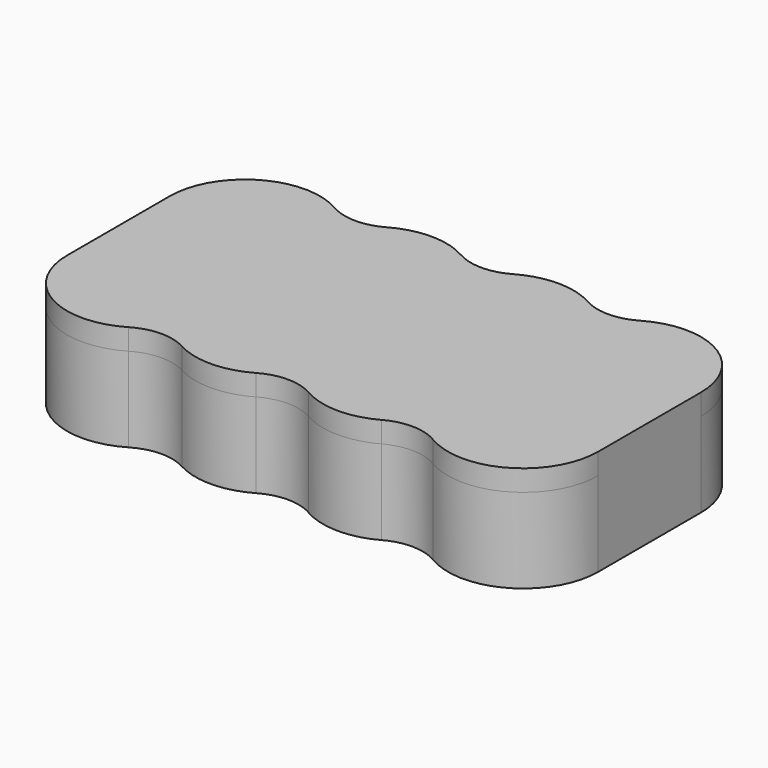
from build123d import *

# Parameters (mm, degrees)
F1_DEPTH  = 8
F2_R      = 5
F3_R      = 5.1
F5_DEPTH  = 2
F6_R      = 2
F7_DEPTH  = 1.5
F8_R      = 1.49999
F9_R      = 2
F10_DEPTH = 1.5
F11_R     = 1.49999


# Not quite as in the source:
# - a fillet or chamfer is up to 0.001 mm smaller than in the source, because OpenCascade refuses the exact size


with BuildPart() as f1:
    # F0 (on Top) → F1 (new body)
    with BuildSketch(Plane.XY):
        with BuildLine():
            ThreePointArc((0, 9.7960505792), (-5.9794748492, 13.0999703322), (-11.9779520569, 9.830677382))
            ThreePointArc((-11.9779520569, 9.830677382), (-19.9562029041, 12.8948954194), (-25.1, 6.0697016347))
            Line((-25.1, 6.0697016347), (-25.1, -6.0697016347))
            ThreePointArc((-25.1, -6.0697016347), (-19.9296547743, -12.9024486996), (-11.9488922671, -9.7837419151))
            ThreePointArc((-11.9488922671, -9.7837419151), (-5.9300692346, -12.9669396851), (0, -9.6213070677))
            ThreePointArc((0, -9.6213070677), (5.9300692346, -12.9669396851), (11.9488922671, -9.7837419151))
            ThreePointArc((11.9488922671, -9.7837419151), (19.9296547743, -12.9024486996), (25.1, -6.0697016347))
            Line((25.1, -6.0697016347), (25.1, 6.0697016347))
            ThreePointArc((25.1, 6.0697016347), (19.9562029041, 12.8948954194), (11.9779520569, 9.830677382))
            ThreePointArc((11.9779520569, 9.830677382), (5.9794748492, 13.0999703322), (0, 9.7960505792))
        make_face()
        with BuildLine():
            ThreePointArc((-24.1, 6.0697016347), (-18.5343432382, 12.1462530666), (-11.9936139988, 7.1342800509))
            ThreePointArc((-11.9936139988, 7.1342800509), (-5.9825651004, 12.0999750839), (0, 7.1))
            ThreePointArc((0, 7.1), (5.9825651004, 12.0999750839), (11.9936139988, 7.1342800509))
            ThreePointArc((11.9936139988, 7.1342800509), (18.5343432382, 12.1462530666), (24.1, 6.0697016347))
            Line((24.1, 6.0697016347), (24.1, -6.0697016347))
            ThreePointArc((24.1, -6.0697016347), (18.5343432382, -12.1462530666), (11.9936139988, -7.1342800509))
            ThreePointArc((11.9936139988, -7.1342800509), (5.8623077698, -11.9653833554), (0, -6.8111789722))
            ThreePointArc((0, -6.8111789722), (-5.8623077698, -11.9653833554), (-11.9936139988, -7.1342800509))
            ThreePointArc((-11.9936139988, -7.1342800509), (-18.5343432382, -12.1462530666), (-24.1, -6.0697016347))
            Line((-24.1, -6.0697016347), (-24.1, 6.0697016347))
        make_face(mode=Mode.SUBTRACT)
    extrude(amount=F1_DEPTH)

    # F2
    f2_edges = [f1.edges().sort_by_distance(p)[0] for p in [
        (-11.948892, -9.783742, 4),
        (0, -9.621307, 4),
        (11.948892, -9.783742, 4),
        (-11.977952, 9.830677, 4),
        (0, 9.796051, 4),
        (11.977952, 9.830677, 4),
    ]]
    fillet(f2_edges, radius=F2_R)

    # F3
    f3_edges = [f1.edges().sort_by_distance(p)[0] for p in [
        (-11.993614, -7.13428, 4),
        (0, -6.811179, 4),
        (11.993614, -7.13428, 4),
        (11.993614, 7.13428, 4),
        (0, 7.1, 4),
        (-11.993614, 7.13428, 4),
    ]]
    fillet(f3_edges, radius=F3_R)

    # F4 (on face) → F5 (join)
    with BuildSketch(Plane.XY.offset(8)):
        with BuildLine():
            ThreePointArc((-9.4848491067, 12.1859378193), (-11.9680100538, 11.5423164018), (-14.4435267926, 12.2147401477))
            ThreePointArc((-14.4435267926, 12.2147401477), (-21.5467619195, 12.2203503717), (-25.1, 6.0697016347))
            Line((-25.1, 6.0697016347), (-25.1, -6.0697016347))
            ThreePointArc((-25.1, -6.0697016347), (-21.5163446166, -12.2377905233), (-14.3830082993, -12.179314637))
            ThreePointArc((-14.3830082993, -12.179314637), (-11.9202167891, -11.4825711508), (-9.4353135356, -12.0957997614))
            ThreePointArc((-9.4353135356, -12.0957997614), (-5.9534768613, -12.9672192968), (-2.4903217652, -12.0242901298))
            ThreePointArc((-2.4903217652, -12.0242901298), (0, -11.3599904776), (2.4903217652, -12.0242901298))
            ThreePointArc((2.4903217652, -12.0242901298), (5.9534768613, -12.9672192968), (9.4353135356, -12.0957997614))
            ThreePointArc((9.4353135356, -12.0957997614), (11.9202167891, -11.4825711508), (14.3830082993, -12.179314637))
            ThreePointArc((14.3830082993, -12.179314637), (21.5163446166, -12.2377905233), (25.1, -6.0697016347))
            Line((25.1, -6.0697016347), (25.1, 6.0697016347))
            ThreePointArc((25.1, 6.0697016347), (21.5467619195, 12.2203503717), (14.4435267926, 12.2147401477))
            ThreePointArc((14.4435267926, 12.2147401477), (11.9680100538, 11.5423164018), (9.4848491067, 12.1859378193))
            ThreePointArc((9.4848491067, 12.1859378193), (5.9794143891, 13.0999701572), (2.479338843, 12.1656260848))
            ThreePointArc((2.479338843, 12.1656260848), (0, 11.5076162853), (-2.479338843, 12.1656260848))
            ThreePointArc((-2.479338843, 12.1656260848), (-5.9794143891, 13.0999701572), (-9.4848491067, 12.1859378193))
        make_face()
    extrude(amount=F5_DEPTH)

    # F6 (on face) → F7 (join)
    with BuildSketch(Plane.YZ.offset(-24.1)):
        with Locations((0, 4)):
            Circle(F6_R)
    extrude(amount=F7_DEPTH)

    # F8 (radius 1.5 in the source; OpenCascade refuses exactly that, so slightly less here)
    f8_edges = [f1.edges().sort_by_distance(p)[0] for p in [
        (-22.6, -2, 4),
    ]]
    fillet(f8_edges, radius=F8_R)

    # F9 (on face) → F10 (join)
    with BuildSketch(Plane(origin=(24.1, 0, 0), x_dir=(0, -1, 0), z_dir=(-1, 0, 0))):
        with Locations((0, 4)):
            Circle(F9_R)
    extrude(amount=F10_DEPTH)

    # F11 (radius 1.5 in the source; OpenCascade refuses exactly that, so slightly less here)
    f11_edges = [f1.edges().sort_by_distance(p)[0] for p in [
        (22.6, 2, 4),
    ]]
    fillet(f11_edges, radius=F11_R)


solid = f1.part
